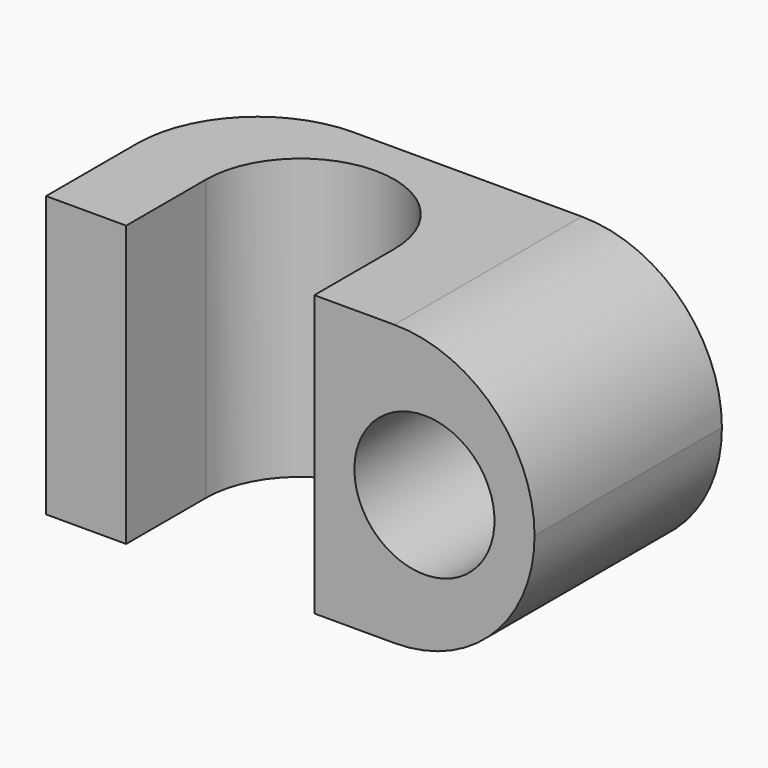
from build123d import *

# Parameters (mm, degrees)
F1_DEPTH = 7
F2_R     = 1.75
F3_DEPTH = 5.85
F4_R     = 3.49999
F5_R     = 3


# Not quite as in the source:
# - a fillet or chamfer is up to 0.001 mm smaller than in the source, because OpenCascade refuses the exact size


with BuildPart() as f1:
    # F0 (on Top) → F1 (new body)
    with BuildSketch(Plane.XY):
        with BuildLine():
            ThreePointArc((-2.35, 0), (0, 2.35), (2.35, 0))
            Line((2.35, 0), (2.35, -2.5))
            Line((2.35, -2.5), (7.85, -2.5))
            Line((7.85, -2.5), (7.85, 3.35))
            Line((7.85, 3.35), (-4.35, 3.35))
            Line((-4.35, 3.35), (-4.35, -2.5))
            Line((-4.35, -2.5), (-2.35, -2.5))
            Line((-2.35, -2.5), (-2.35, 0))
        make_face()
    extrude(amount=F1_DEPTH)

    # F2 (on face) → F3 (cut, through all)
    with BuildSketch(Plane(origin=(0, 3.35, 0), x_dir=(-1, 0, 0), z_dir=(0, 1, 0))):
        with Locations((-5.1, 3.5)):
            Circle(F2_R)
    extrude(amount=-F3_DEPTH, mode=Mode.SUBTRACT)

    # F4 (radius 3.5 in the source; OpenCascade refuses exactly that, so slightly less here)
    f4_edges = [f1.edges().sort_by_distance(p)[0] for p in [
        (7.85, 0.425, 7),
        (7.85, 0.425, 0),
    ]]
    fillet(f4_edges, radius=F4_R)

    # F5
    f5_edges = [f1.edges().sort_by_distance(p)[0] for p in [
        (-4.35, 3.35, 3.5),
    ]]
    fillet(f5_edges, radius=F5_R)


solid = f1.part
